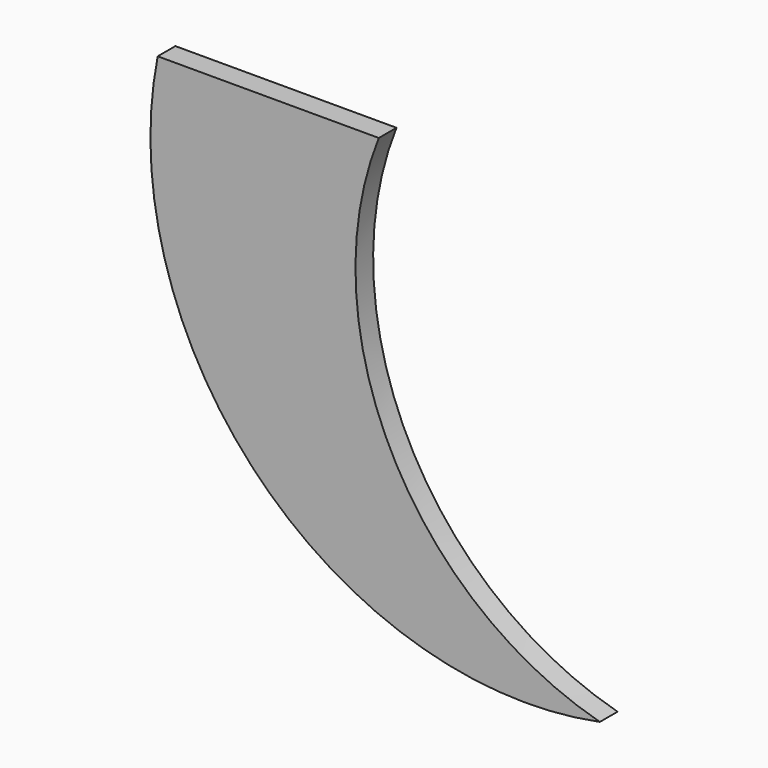
from build123d import *

# Parameters (mm, degrees)
F1_DEPTH = 25


# Not quite as in the source:
# - a feature names something its author has since deleted; it is built from what else it names


with BuildPart() as f1:
    # F0 (on Front) → F1 (new body)
    with BuildSketch(Plane.XZ):
        with BuildLine():
            Line((250, 0), (0, 0))
            ThreePointArc((0, 0), (116.2504187973, -383.7495812027), (500, -500))
            ThreePointArc((500, -500), (263.196601125, -305.9016994375), (250, 0))
        make_face()
    extrude(amount=F1_DEPTH)


solid = f1.part
